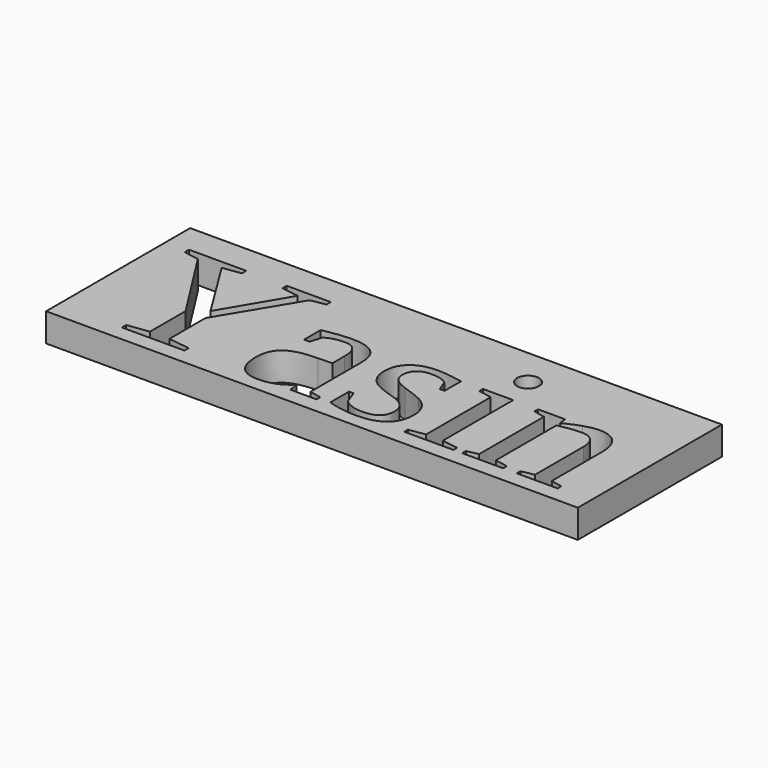
from build123d import *

# Parameters (mm, degrees)
F0_W     = 75
F0_H     = 25.4
F1_DEPTH = 4


with BuildPart() as f1:
    # F0 (on Top) → F1 (new body)
    with BuildSketch(Plane.XY):
        with Locations((61.0273839791, -20.1516905552)):
            Rectangle(F0_W, F0_H)
        Polygon((44.541381375, -12.6777322218), (38.2477615833, -23.1321593052), (38.2477615833, -29.5123676385), (41.2783605416, -29.8951801385), (41.2783605416, -30.6516905552), (32.4645584583, -30.6516905552), (32.4645584583, -29.8951801385), (35.4997147083, -29.5123676385), (35.4997147083, -23.2187478468), (28.791381375, -12.6777322218), (26.6403397083, -12.3085915968), (26.6403397083, -11.5520811802), (34.7158605416, -11.5520811802), (34.7158605416, -12.3085915968), (32.1501053333, -12.6777322218), (37.6325272083, -21.4960915968), (42.846068875, -12.6777322218), (40.426147, -12.3085915968), (40.426147, -11.5520811802), (46.63317825, -11.5520811802), (46.63317825, -12.3085915968), align=None, mode=Mode.SUBTRACT)
        with BuildLine():
            add(Edge.make_bspline(
                [(49.941772, -17.4628884718), (52.2477615833, -16.9661436802), (53.9977615833, -16.9661436802)],
                knots=[0, 0, 0, 1, 1, 1], degree=2))
            add(Edge.make_bspline(
                [(53.9977615833, -16.9661436802), (56.189818875, -16.9661436802), (57.2243240833, -17.8639301385)],
                knots=[0, 0, 0, 1, 1, 1], degree=2))
            add(Edge.make_bspline(
                [(57.2243240833, -17.8639301385), (58.2588292916, -18.7617165968), (58.2588292916, -20.6119770135)],
                knots=[0, 0, 0, 1, 1, 1], degree=2))
            Line((58.2588292916, -20.6119770135), (58.2588292916, -29.6536436802))
            Line((58.2588292916, -29.6536436802), (59.92224075, -30.0091124302))
            Line((59.92224075, -30.0091124302), (59.92224075, -30.6516905552))
            Line((59.92224075, -30.6516905552), (56.2490636666, -30.6516905552))
            Line((56.2490636666, -30.6516905552), (55.9801834583, -29.3118468052))
            add(Edge.make_bspline(
                [(55.9801834583, -29.3118468052), (54.3532303333, -30.9387999302), (51.8330480416, -30.9387999302)],
                knots=[0, 0, 0, 1, 1, 1], degree=2))
            add(Edge.make_bspline(
                [(51.8330480416, -30.9387999302), (48.4014074166, -30.9387999302), (48.4014074166, -26.9466124302)],
                knots=[0, 0, 0, 1, 1, 1], degree=2))
            add(Edge.make_bspline(
                [(48.4014074166, -26.9466124302), (48.4014074166, -25.6113259718), (48.9209386666, -24.734047326)],
                knots=[0, 0, 0, 1, 1, 1], degree=2))
            add(Edge.make_bspline(
                [(48.9209386666, -24.734047326), (49.4404699166, -23.8567686802), (50.5797928333, -23.394203576)],
                knots=[0, 0, 0, 1, 1, 1], degree=2))
            add(Edge.make_bspline(
                [(50.5797928333, -23.394203576), (51.71911575, -22.9316384718), (53.8838292916, -22.8906228468)],
                knots=[0, 0, 0, 1, 1, 1], degree=2))
            Line((53.8838292916, -22.8906228468), (55.8935949166, -22.8313780552))
            Line((55.8935949166, -22.8313780552), (55.8935949166, -20.7395811802))
            add(Edge.make_bspline(
                [(55.8935949166, -20.7395811802), (55.8935949166, -19.3587218052), (55.3877355416, -18.7024718052)],
                knots=[0, 0, 0, 1, 1, 1], degree=2))
            add(Edge.make_bspline(
                [(55.3877355416, -18.7024718052), (54.8818761666, -18.0462218052), (53.8291417916, -18.0462218052)],
                knots=[0, 0, 0, 1, 1, 1], degree=2))
            add(Edge.make_bspline(
                [(53.8291417916, -18.0462218052), (52.4027095, -18.0462218052), (51.2223709583, -18.7161436802)],
                knots=[0, 0, 0, 1, 1, 1], degree=2))
            Line((51.2223709583, -18.7161436802), (50.7392980416, -20.3841124302))
            Line((50.7392980416, -20.3841124302), (49.941772, -20.3841124302))
            Line((49.941772, -20.3841124302), (49.941772, -17.4628884718))
        make_face(mode=Mode.SUBTRACT)
        with BuildLine():
            add(Edge.make_bspline(
                [(70.3698318958, -25.3811827427), (70.6182042916, -25.9941384718), (70.6182042916, -26.8919249302)],
                knots=[0, 0, 0, 1, 1, 1], degree=2))
            add(Edge.make_bspline(
                [(70.6182042916, -26.8919249302), (70.6182042916, -28.8834613885), (69.3581131458, -29.9111306593)],
                knots=[0, 0, 0, 1, 1, 1], degree=2))
            add(Edge.make_bspline(
                [(69.3581131458, -29.9111306593), (68.098022, -30.9387999302), (65.6370845, -30.9387999302)],
                knots=[0, 0, 0, 1, 1, 1], degree=2))
            add(Edge.make_bspline(
                [(65.6370845, -30.9387999302), (64.639037625, -30.9387999302), (63.435912625, -30.7314431593)],
                knots=[0, 0, 0, 1, 1, 1], degree=2))
            add(Edge.make_bspline(
                [(63.435912625, -30.7314431593), (62.232787625, -30.5240863885), (61.549193875, -30.2688780552)],
                knots=[0, 0, 0, 1, 1, 1], degree=2))
            Line((61.549193875, -30.2688780552), (61.549193875, -26.9785134718))
            Line((61.549193875, -26.9785134718), (62.1872147083, -26.9785134718))
            Line((62.1872147083, -26.9785134718), (62.889037625, -28.8424457635))
            add(Edge.make_bspline(
                [(62.889037625, -28.8424457635), (63.955443875, -29.8131488885), (65.66442825, -29.8131488885)],
                knots=[0, 0, 0, 1, 1, 1], degree=2))
            add(Edge.make_bspline(
                [(65.66442825, -29.8131488885), (68.426147, -29.8131488885), (68.426147, -27.4479145135)],
                knots=[0, 0, 0, 1, 1, 1], degree=2))
            add(Edge.make_bspline(
                [(68.426147, -27.4479145135), (68.426147, -25.7115863885), (66.2477615833, -24.9687478468)],
                knots=[0, 0, 0, 1, 1, 1], degree=2))
            Line((66.2477615833, -24.9687478468), (64.9808345, -24.5540343052))
            add(Edge.make_bspline(
                [(64.9808345, -24.5540343052), (63.5407303333, -24.0846332635), (62.8867589791, -23.6015603468)],
                knots=[0, 0, 0, 1, 1, 1], degree=2))
            add(Edge.make_bspline(
                [(62.8867589791, -23.6015603468), (62.232787625, -23.1184874302), (61.877318875, -22.4121072218)],
                knots=[0, 0, 0, 1, 1, 1], degree=2))
            add(Edge.make_bspline(
                [(61.877318875, -22.4121072218), (61.521850125, -21.7057270135), (61.521850125, -20.7122374302)],
                knots=[0, 0, 0, 1, 1, 1], degree=2))
            add(Edge.make_bspline(
                [(61.521850125, -20.7122374302), (61.521850125, -18.9440082635), (62.724975125, -17.925453576)],
                knots=[0, 0, 0, 1, 1, 1], degree=2))
            add(Edge.make_bspline(
                [(62.724975125, -17.925453576), (63.928100125, -16.9068988885), (65.978881375, -16.9068988885)],
                knots=[0, 0, 0, 1, 1, 1], degree=2))
            add(Edge.make_bspline(
                [(65.978881375, -16.9068988885), (67.4463292916, -16.9068988885), (69.6520584583, -17.3489561802)],
                knots=[0, 0, 0, 1, 1, 1], degree=2))
            Line((69.6520584583, -17.3489561802), (69.6520584583, -20.2701801385))
            Line((69.6520584583, -20.2701801385), (68.9821365833, -20.2701801385))
            Line((68.9821365833, -20.2701801385), (68.385131375, -18.7161436802))
            add(Edge.make_bspline(
                [(68.385131375, -18.7161436802), (67.6286209583, -18.0462218052), (66.006225125, -18.0462218052)],
                knots=[0, 0, 0, 1, 1, 1], degree=2))
            add(Edge.make_bspline(
                [(66.006225125, -18.0462218052), (64.8532303333, -18.0462218052), (64.2471105416, -18.6158832635)],
                knots=[0, 0, 0, 1, 1, 1], degree=2))
            add(Edge.make_bspline(
                [(64.2471105416, -18.6158832635), (63.64099075, -19.1855447218), (63.64099075, -20.1562478468)],
                knots=[0, 0, 0, 1, 1, 1], degree=2))
            add(Edge.make_bspline(
                [(63.64099075, -20.1562478468), (63.64099075, -20.9674457635), (64.1901443958, -21.5234353468)],
                knots=[0, 0, 0, 1, 1, 1], degree=2))
            add(Edge.make_bspline(
                [(64.1901443958, -21.5234353468), (64.7392980416, -22.0794249302), (65.8512772083, -22.4485655552)],
                knots=[0, 0, 0, 1, 1, 1], degree=2))
            add(Edge.make_bspline(
                [(65.8512772083, -22.4485655552), (67.9430740833, -23.1595030552), (68.5833735625, -23.4876280552)],
                knots=[0, 0, 0, 1, 1, 1], degree=2))
            add(Edge.make_bspline(
                [(68.5833735625, -23.4876280552), (69.2236730416, -23.8157530552), (69.6725662708, -24.2919900343)],
                knots=[0, 0, 0, 1, 1, 1], degree=2))
            add(Edge.make_bspline(
                [(69.6725662708, -24.2919900343), (70.1214595, -24.7682270135), (70.3698318958, -25.3811827427)],
                knots=[0, 0, 0, 1, 1, 1], degree=2))
        make_face(mode=Mode.SUBTRACT)
        Polygon((76.93005325, -17.2623676385), (76.93005325, -29.6536436802), (79.2223709583, -30.0091124302), (79.2223709583, -30.6516905552), (72.2861730416, -30.6516905552), (72.2861730416, -30.0091124302), (74.564818875, -29.6536436802), (74.564818875, -18.2604145135), (72.6735428333, -17.9049457635), (72.6735428333, -17.2623676385), align=None, mode=Mode.SUBTRACT)
        with BuildLine():
            Line((84.2627355416, -17.2623676385), (84.394897, -18.3470030552))
            add(Edge.make_bspline(
                [(84.394897, -18.3470030552), (85.488647, -17.7180968052), (86.7282303333, -17.3124978468)],
                knots=[0, 0, 0, 1, 1, 1], degree=2))
            add(Edge.make_bspline(
                [(86.7282303333, -17.3124978468), (87.9678136666, -16.9068988885), (88.7926834583, -16.9068988885)],
                knots=[0, 0, 0, 1, 1, 1], degree=2))
            add(Edge.make_bspline(
                [(88.7926834583, -16.9068988885), (90.5290115833, -16.9068988885), (91.4131261666, -17.9186176385)],
                knots=[0, 0, 0, 1, 1, 1], degree=2))
            add(Edge.make_bspline(
                [(91.4131261666, -17.9186176385), (92.29724075, -18.9303363885), (92.29724075, -20.8535134718)],
                knots=[0, 0, 0, 1, 1, 1], degree=2))
            Line((92.29724075, -20.8535134718), (92.29724075, -29.6536436802))
            Line((92.29724075, -29.6536436802), (93.9196365833, -30.0091124302))
            Line((93.9196365833, -30.0091124302), (93.9196365833, -30.6516905552))
            Line((93.9196365833, -30.6516905552), (88.154662625, -30.6516905552))
            Line((88.154662625, -30.6516905552), (88.154662625, -30.0091124302))
            Line((88.154662625, -30.0091124302), (89.932006375, -29.6536436802))
            Line((89.932006375, -29.6536436802), (89.932006375, -21.1087218052))
            add(Edge.make_bspline(
                [(89.932006375, -21.1087218052), (89.932006375, -19.9283832635), (89.3555089791, -19.251625451)],
                knots=[0, 0, 0, 1, 1, 1], degree=2))
            add(Edge.make_bspline(
                [(89.3555089791, -19.251625451), (88.7790115833, -18.5748676385), (87.566772, -18.5748676385)],
                knots=[0, 0, 0, 1, 1, 1], degree=2))
            add(Edge.make_bspline(
                [(87.566772, -18.5748676385), (86.2861730416, -18.5748676385), (84.42224075, -18.9895811802)],
                knots=[0, 0, 0, 1, 1, 1], degree=2))
            Line((84.42224075, -18.9895811802), (84.42224075, -29.6536436802))
            Line((84.42224075, -29.6536436802), (86.2314855416, -30.0091124302))
            Line((86.2314855416, -30.0091124302), (86.2314855416, -30.6516905552))
            Line((86.2314855416, -30.6516905552), (80.4482824166, -30.6516905552))
            Line((80.4482824166, -30.6516905552), (80.4482824166, -30.0091124302))
            Line((80.4482824166, -30.0091124302), (82.057006375, -29.6536436802))
            Line((82.057006375, -29.6536436802), (82.057006375, -18.2604145135))
            Line((82.057006375, -18.2604145135), (80.4482824166, -17.9049457635))
            Line((80.4482824166, -17.9049457635), (80.4482824166, -17.2623676385))
            Line((80.4482824166, -17.2623676385), (84.2627355416, -17.2623676385))
        make_face(mode=Mode.SUBTRACT)
        with BuildLine():
            add(Edge.make_bspline(
                [(76.615600125, -11.7936176385), (77.0713292916, -12.2493468052), (77.0713292916, -12.8919249302)],
                knots=[0, 0, 0, 1, 1, 1], degree=2))
            add(Edge.make_bspline(
                [(77.0713292916, -12.8919249302), (77.0713292916, -13.5208311802), (76.615600125, -13.9765603468)],
                knots=[0, 0, 0, 1, 1, 1], degree=2))
            add(Edge.make_bspline(
                [(76.615600125, -13.9765603468), (76.1598709583, -14.4322895135), (75.521850125, -14.4322895135)],
                knots=[0, 0, 0, 1, 1, 1], degree=2))
            add(Edge.make_bspline(
                [(75.521850125, -14.4322895135), (74.892943875, -14.4322895135), (74.4372147083, -13.9765603468)],
                knots=[0, 0, 0, 1, 1, 1], degree=2))
            add(Edge.make_bspline(
                [(74.4372147083, -13.9765603468), (73.9814855416, -13.5208311802), (73.9814855416, -12.8919249302)],
                knots=[0, 0, 0, 1, 1, 1], degree=2))
            add(Edge.make_bspline(
                [(73.9814855416, -12.8919249302), (73.9814855416, -12.2493468052), (74.4372147083, -11.7936176385)],
                knots=[0, 0, 0, 1, 1, 1], degree=2))
            add(Edge.make_bspline(
                [(74.4372147083, -11.7936176385), (74.892943875, -11.3378884718), (75.521850125, -11.3378884718)],
                knots=[0, 0, 0, 1, 1, 1], degree=2))
            add(Edge.make_bspline(
                [(75.521850125, -11.3378884718), (76.1598709583, -11.3378884718), (76.615600125, -11.7936176385)],
                knots=[0, 0, 0, 1, 1, 1], degree=2))
        make_face(mode=Mode.SUBTRACT)
    extrude(amount=F1_DEPTH)


solid = f1.part
